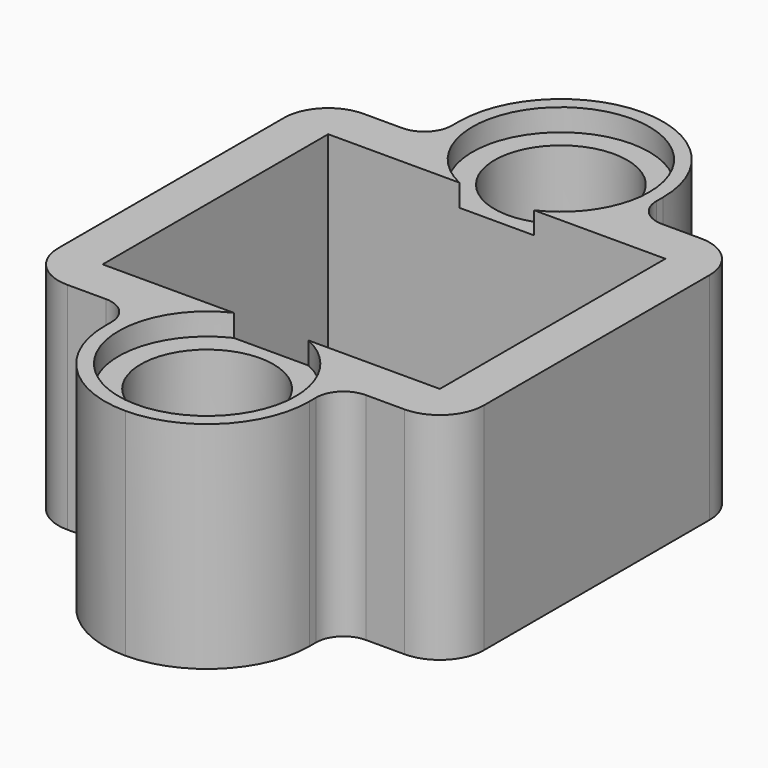
from build123d import *

# Parameters (mm, degrees)
F1_DEPTH = 7.8
F2_START = 0.8
F0_R     = 2.4
F2_DEPTH = 6.2
F0_R_2   = 1
F0_R_3   = 2
F3_DEPTH = 0.8


# Not quite as in the source:
# - a feature names something its author has since deleted; it is built from what else it names


with BuildPart() as f1:
    # F0 (on Top) → F1 (new body)
    with BuildSketch(Plane.XY):
        with BuildLine():
            ThreePointArc((0, 11.7), (-2.6162950904, 10.6162950904), (-3.7, 8))
            Line((-3.7, 8), (-3.7, 7.7))
            ThreePointArc((-3.7, 7.7), (-3.9928932188, 6.9928932188), (-4.7, 6.7))
            Line((-4.7, 6.7), (-6.1, 6.7))
            ThreePointArc((-6.1, 6.7), (-7.2313708499, 6.2313708499), (-7.7, 5.1))
            Line((-7.7, 5.1), (-7.7, -5.1))
            ThreePointArc((-7.7, -5.1), (-7.2313708499, -6.2313708499), (-6.1, -6.7))
            Line((-6.1, -6.7), (-4.7, -6.7))
            ThreePointArc((-4.7, -6.7), (-3.9928932188, -6.9928932188), (-3.7, -7.7))
            Line((-3.7, -7.7), (-3.7, -8))
            ThreePointArc((-3.7, -8), (-2.6162950904, -10.6162950904), (0, -11.7))
            ThreePointArc((0, -11.7), (2.6162950904, -10.6162950904), (3.7, -8))
            Line((3.7, -8), (3.7, -7.7))
            ThreePointArc((3.7, -7.7), (3.9928932188, -6.9928932188), (4.7, -6.7))
            Line((4.7, -6.7), (6.1, -6.7))
            ThreePointArc((6.1, -6.7), (7.2313708499, -6.2313708499), (7.7, -5.1))
            Line((7.7, -5.1), (7.7, 5.1))
            ThreePointArc((7.7, 5.1), (7.2313708499, 6.2313708499), (6.1, 6.7))
            Line((6.1, 6.7), (4.7, 6.7))
            ThreePointArc((4.7, 6.7), (3.9928932188, 6.9928932188), (3.7, 7.7))
            Line((3.7, 7.7), (3.7, 8))
            ThreePointArc((3.7, 8), (2.6162950904, 10.6162950904), (0, 11.7))
        make_face()
        with BuildLine():
            Line((-6.1, -5.1), (-6.1, 5.1))
            Line((-6.1, 5.1), (-1.3527749258, 5.1))
            ThreePointArc((-1.3527749258, 5.1), (-1.7191742549, 10.698970152), (3.2, 8))
            ThreePointArc((3.2, 8), (2.698970152, 6.2808257451), (1.3527749258, 5.1))
            Line((1.3527749258, 5.1), (6.1, 5.1))
            Line((6.1, 5.1), (6.1, -5.1))
            Line((6.1, -5.1), (1.3527749258, -5.1))
            ThreePointArc((1.3527749258, -5.1), (2.698970152, -6.2808257451), (3.2, -8))
            ThreePointArc((3.2, -8), (-1.7191742549, -10.698970152), (-1.3527749258, -5.1))
            Line((-1.3527749258, -5.1), (-6.1, -5.1))
        make_face(mode=Mode.SUBTRACT)
    extrude(amount=F1_DEPTH)

    # F0 (on Top) → F2 (join)
    with BuildSketch(Plane.XY.offset(F2_START)):
        with BuildLine():
            Line((1.3527749258, -5.1), (-1.3527749258, -5.1))
            ThreePointArc((-1.3527749258, -5.1), (-1.7191742549, -10.698970152), (3.2, -8))
            ThreePointArc((3.2, -8), (2.698970152, -6.2808257451), (1.3527749258, -5.1))
        make_face()
        with Locations((0, -8)):
            Circle(F0_R, mode=Mode.SUBTRACT)
        with BuildLine():
            ThreePointArc((3.2, 8), (-1.7191742549, 10.698970152), (-1.3527749258, 5.1))
            Line((-1.3527749258, 5.1), (1.3527749258, 5.1))
            ThreePointArc((1.3527749258, 5.1), (2.698970152, 6.2808257451), (3.2, 8))
        make_face()
        with Locations((0, 8)):
            Circle(F0_R, mode=Mode.SUBTRACT)
    extrude(amount=F2_DEPTH)

    # F0 (on Top) → F3 (join)
    with BuildSketch(Plane.XY):
        with BuildLine():
            Line((-1.3527749258, 5.1), (-6.1, 5.1))
            Line((-6.1, 5.1), (-6.1, -5.1))
            Line((-6.1, -5.1), (-1.3527749258, -5.1))
            ThreePointArc((-1.3527749258, -5.1), (0, -4.8), (1.3527749258, -5.1))
            Line((1.3527749258, -5.1), (6.1, -5.1))
            Line((6.1, -5.1), (6.1, 5.1))
            Line((6.1, 5.1), (1.3527749258, 5.1))
            ThreePointArc((1.3527749258, 5.1), (0, 4.8), (-1.3527749258, 5.1))
        make_face()
        with Locations((-4.5, 0)):
            Circle(F0_R_2, mode=Mode.SUBTRACT)
        Circle(F0_R_3, mode=Mode.SUBTRACT)
        with Locations((4.5, 0)):
            Circle(F0_R_2, mode=Mode.SUBTRACT)
    extrude(amount=F3_DEPTH)


solid = f1.part
